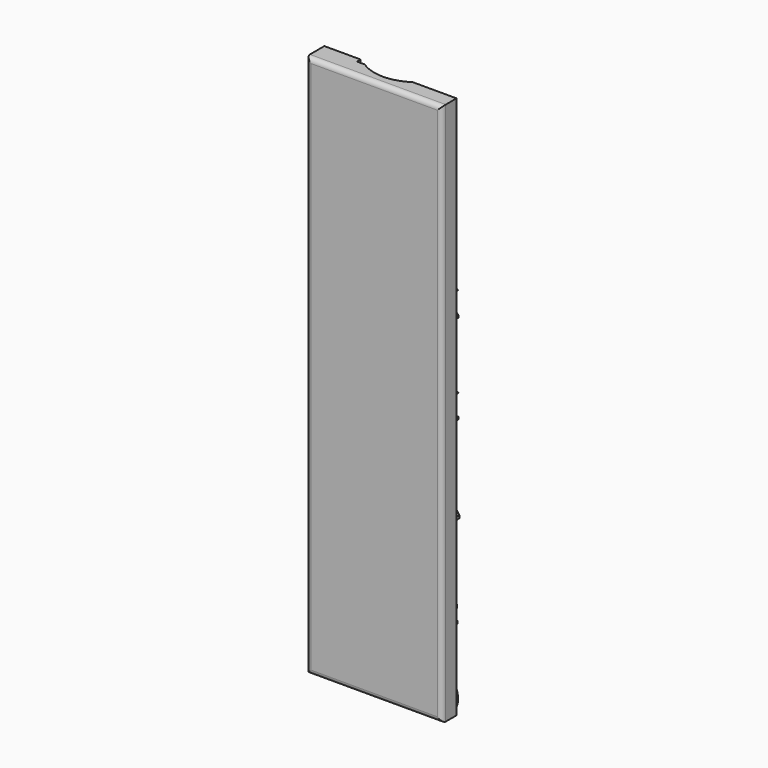
from build123d import *

# Parameters (mm, degrees)
F1_DEPTH     = 60
F2_R         = 0.508
F3_W         = 4
F3_H         = 0.5
F3_H_2       = 1
F3_W_2       = 3
F4_DEPTH     = 0.5
F5_TEXT_SIZE = 4.1884917792
F6_DEPTH     = 0.5


# Not quite as in the source:
# - Text() gives the source's letters only with a copy of the font that has no kerning and outlines rounded to 1/6400 em; it was checked with that copy


with BuildPart() as f1:
    # F0 (on Top) → F1 (new body)
    with BuildSketch(Plane.XY):
        with BuildLine():
            Line((0, 2), (0, 0))
            Line((0, 0), (15, 0))
            Line((15, 0), (15, 2))
            Line((15, 2), (10.1472396027, 2))
            ThreePointArc((10.1472396027, 2), (7.5, 1.1939348988), (4.8527603973, 2))
            Line((4.8527603973, 2), (0, 2))
        make_face()
    extrude(amount=-F1_DEPTH)

    # F2
    f2_edges = [f1.edges().sort_by_distance(p)[0] for p in [
        (0, 0, -30),
        (15, 0, -30),
        (7.5, 0, 0),
        (7.5, 0, -60),
    ]]
    fillet(f2_edges, radius=F2_R)

    # F3 (on face) → F4 (join)
    with BuildSketch(Plane(origin=(0, 2, 0), x_dir=(-1, 0, 0), z_dir=(0, 1, 0))):
        with Locations((-2, -0.25)):
            Rectangle(F3_W, F3_H)
        with Locations((-2, -10)):
            Rectangle(F3_W, F3_H_2)
        with Locations((-1.5, -5)):
            Rectangle(F3_W_2, F3_H_2)
        with Locations((-1.5, -15)):
            Rectangle(F3_W_2, F3_H_2)
        with Locations((-2, -20)):
            Rectangle(F3_W, F3_H_2)
        with Locations((-1.5, -25)):
            Rectangle(F3_W_2, F3_H_2)
        with Locations((-2, -30)):
            Rectangle(F3_W, F3_H_2)
        with Locations((-1.5, -35)):
            Rectangle(F3_W_2, F3_H_2)
        with Locations((-2, -40)):
            Rectangle(F3_W, F3_H_2)
        with Locations((-1.5, -45)):
            Rectangle(F3_W_2, F3_H_2)
        with Locations((-2, -50)):
            Rectangle(F3_W, F3_H_2)
        with Locations((-1.5, -55)):
            Rectangle(F3_W_2, F3_H_2)
        with Locations((-2, -59.75)):
            Rectangle(F3_W, F3_H)
    extrude(amount=F4_DEPTH)

    # F5 (on face) → F6 (join)
    with BuildSketch(Plane(origin=(0, 2, 0), x_dir=(-1, 0, 0), z_dir=(0, 1, 0))):
        with Locations((-15, -11.5636938991)):
            Text('10', F5_TEXT_SIZE, font='Open Sans', text_align=(TextAlign.LEFT, TextAlign.BOTTOM))
        with Locations((-15, -21.6149968213)):
            Text('20', F5_TEXT_SIZE, font='Open Sans', text_align=(TextAlign.LEFT, TextAlign.BOTTOM))
        with Locations((-15, -31.6214289324)):
            Text('30', F5_TEXT_SIZE, font='Open Sans', text_align=(TextAlign.LEFT, TextAlign.BOTTOM))
        with Locations((-15, -41.7624744084)):
            Text('40', F5_TEXT_SIZE, font='Open Sans', text_align=(TextAlign.LEFT, TextAlign.BOTTOM))
        with Locations((-15, -51.4996704764)):
            Text('50', F5_TEXT_SIZE, font='Open Sans', text_align=(TextAlign.LEFT, TextAlign.BOTTOM))
        with Locations((-15, -60)):
            Text('60', F5_TEXT_SIZE, font='Open Sans', text_align=(TextAlign.LEFT, TextAlign.BOTTOM))
    extrude(amount=F6_DEPTH)


solid = f1.part
